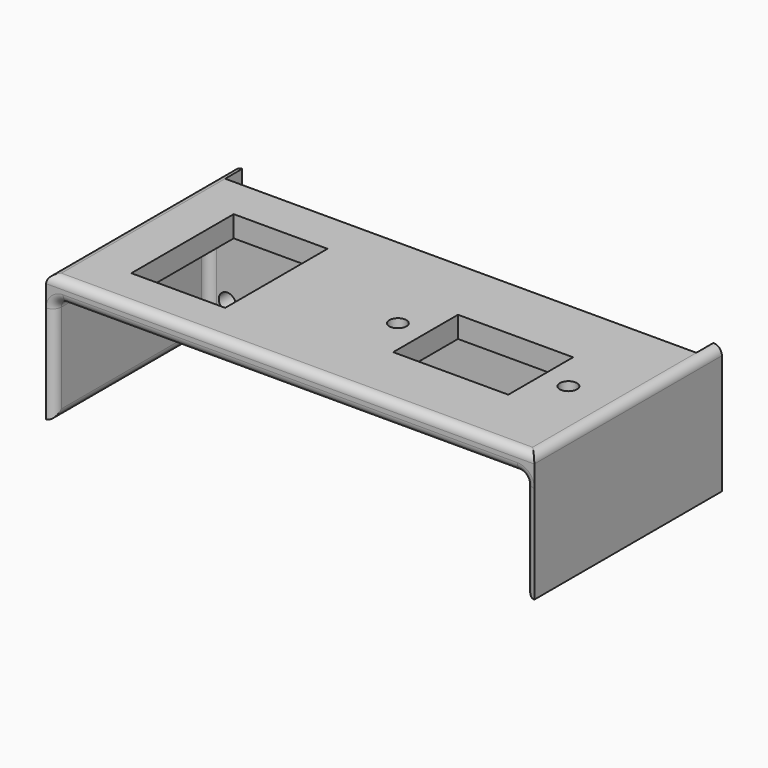
from build123d import *

# Parameters (mm, degrees)
F0_W     = 110.5
F0_H     = 50
F0_W_2   = 22
F0_H_2   = 30
F0_R     = 2
F0_W_3   = 27
F0_H_3   = 19
F1_DEPTH = 5
F2_W     = 110.5
F2_H     = 5
F3_DEPTH = 25
F4_R     = 2
F5_DEPTH = 5.001
F6_W     = 2
F6_H     = 30
F7_DEPTH = 50
F8_DEPTH = 5
F9_F1_R  = 2
F9_F2_R  = 1.9999


# Not quite as in the source:
# - a fillet or chamfer is up to 0.001 mm smaller than in the source, because OpenCascade refuses the exact size


with BuildPart() as f1:
    # F0 (on Top) → F1 (new body)
    with BuildSketch(Plane.XY):
        with Locations((34.25, 0)):
            Rectangle(F0_W, F0_H)
        Rectangle(F0_W_2, F0_H_2, mode=Mode.SUBTRACT)
        with Locations((39.5, 0)):
            Circle(F0_R, mode=Mode.SUBTRACT)
        with Locations((59.5, 0)):
            Rectangle(F0_W_3, F0_H_3, mode=Mode.SUBTRACT)
        with Locations((79.5, 0)):
            Circle(F0_R, mode=Mode.SUBTRACT)
    extrude(amount=F1_DEPTH)

    # F2 (on face) → F3 (join)
    with BuildSketch(Plane(origin=(0, 0, 0), x_dir=(1, 0, 0), z_dir=(0, 0, -1))):
        with Locations((34.25, -22.5)):
            Rectangle(F2_W, F2_H)
    extrude(amount=F3_DEPTH)

    # F4 (on face) → F5 (cut, through all)
    with BuildSketch(Plane.XZ.offset(-20)):
        with Locations((-16.5, -17)):
            Circle(F4_R)
        with Locations((-10.5, -17)):
            Circle(F4_R)
        with Locations((-4.5, -17)):
            Circle(F4_R)
    extrude(amount=-F5_DEPTH, mode=Mode.SUBTRACT)

    # F6 (on face) → F7 (join, through all)
    with BuildSketch(Plane(origin=(0, 25, 0), x_dir=(-1, 0, 0), z_dir=(0, 1, 0))):
        with Locations((22, -10)):
            Rectangle(F6_W, F6_H)
        with Locations((-90.5, -10)):
            Rectangle(F6_W, F6_H)
    extrude(amount=-F7_DEPTH)

    # F6 (on face) → F8 (join)
    with BuildSketch(Plane(origin=(0, 25, 0), x_dir=(-1, 0, 0), z_dir=(0, 1, 0))):
        with Locations((22, -10)):
            Rectangle(F6_W, F6_H)
        with Locations((-90.5, -10)):
            Rectangle(F6_W, F6_H)
    extrude(amount=F8_DEPTH)

    # F9: fillet of radius 2 on 10 edges, made by hand

    # F9_f1
    f9_f1_edges = [f1.edges().sort_by_distance(p)[0] for p in [
        (89.5, 20, -12.5),
        (34.25, 20, 0),
        (89.5, -2.5, 0),
        (-21, 20, -12.5),
        (-21, -2.5, 0),
    ]]
    fillet(f9_f1_edges, radius=F9_F1_R)

    # F9_f2 (radius 2 in the source; OpenCascade refuses exactly that, so slightly less here)
    f9_f2_edges = [f1.edges().sort_by_distance(p)[0] for p in [
        (34.25, -25, 0),
        (34.25, -25, 5),
        (89.5, -3.5, -25),
        (-23, 2.5, 5),
        (91.5, 2.5, 5),
        (88.9142135624, 19.4142135624, -25),
        (-20.4142135624, -25, -0.5857864376),
        (88.9142135624, -25, -0.5857864376),
    ]]
    fillet(f9_f2_edges, radius=F9_F2_R)


solid = f1.part
